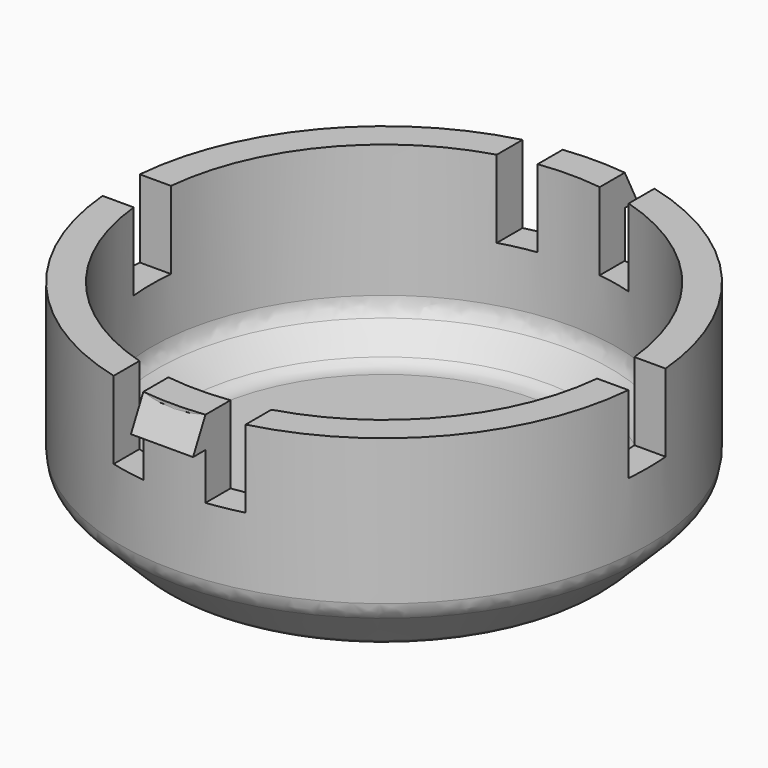
from build123d import *

# Parameters (mm, degrees)
F2_W          = 3
F2_H          = 6.5
F3_DEPTH      = 25
F3_DEPTH_BACK = 25
F4_W          = 2.25
F4_H          = 6.5
F5_DEPTH      = 25
F5_DEPTH_BACK = 25
F6_R          = 1.5
F8_W          = 4
F8_H          = 2
F9_DEPTH      = 1
F10_SIZE2     = 1.99999
F10_SIZE      = 0.99999


# Not quite as in the source:
# - a fillet or chamfer is up to 0.001 mm smaller than in the source, because OpenCascade refuses the exact size


with BuildPart() as f1:
    # F0 (on Front) → F1 (revolve)
    with BuildSketch(Plane.XZ):
        Polygon((0, 2), (0, 0), (13.5, 0), (17, 3.5), (17, 13.5), (15, 13.5), (15, 4.3284271247), (12.6715728753, 2), align=None)
    revolve(axis=Axis((0, 0, 1), (0, 0, -1)))

    # F2 (on Right) → F3 (cut, two sides)
    with BuildSketch(Plane.YZ) as f3_sk:
        with Locations((0, 11.75)):
            Rectangle(F2_W, F2_H)
    extrude(amount=F3_DEPTH, mode=Mode.SUBTRACT)
    extrude(f3_sk.sketch, amount=-F3_DEPTH_BACK, mode=Mode.SUBTRACT)

    # F4 (on Front) → F5 (cut, two sides)
    with BuildSketch(Plane.XZ) as f5_sk:
        with Locations((-3.125, 11.75)):
            Rectangle(F4_W, F4_H)
        with Locations((3.125, 11.75)):
            Rectangle(F4_W, F4_H)
    extrude(amount=F5_DEPTH, mode=Mode.SUBTRACT)
    extrude(f5_sk.sketch, amount=-F5_DEPTH_BACK, mode=Mode.SUBTRACT)

    # F6
    f6_edges = [f1.edges().sort_by_distance(p)[0] for p in [
        (-12.671573, 0, 2),
        (-15, 0, 4.328427),
        (-17, 0, 3.5),
        (-13.5, 0, 0),
    ]]
    fillet(f6_edges, radius=F6_R)

    # F8 (on offset) → F9 (join)
    with BuildSketch(Plane.XZ.offset(16.88)):
        with Locations((0, 12.5)):
            Rectangle(F8_W, F8_H)
    extrude(amount=F9_DEPTH)

    # F10 (size 1 and 2 in the source; OpenCascade refuses exactly that, so slightly less here)
    f10_edges = [f1.edges().sort_by_distance(p)[0] for p in [
        (0, -17.88, 13.5),
    ]]
    f10_side = f1.faces().sort_by_distance((0, -16.417446, 13.5))[0]
    chamfer(f10_edges, length=F10_SIZE, length2=F10_SIZE2, reference=f10_side)

    # F11: F1 across plane


with BuildPart() as f1_1:
    add(f1.part)
    add(f1.part.mirror(Plane.XZ))


solid = f1_1.part
